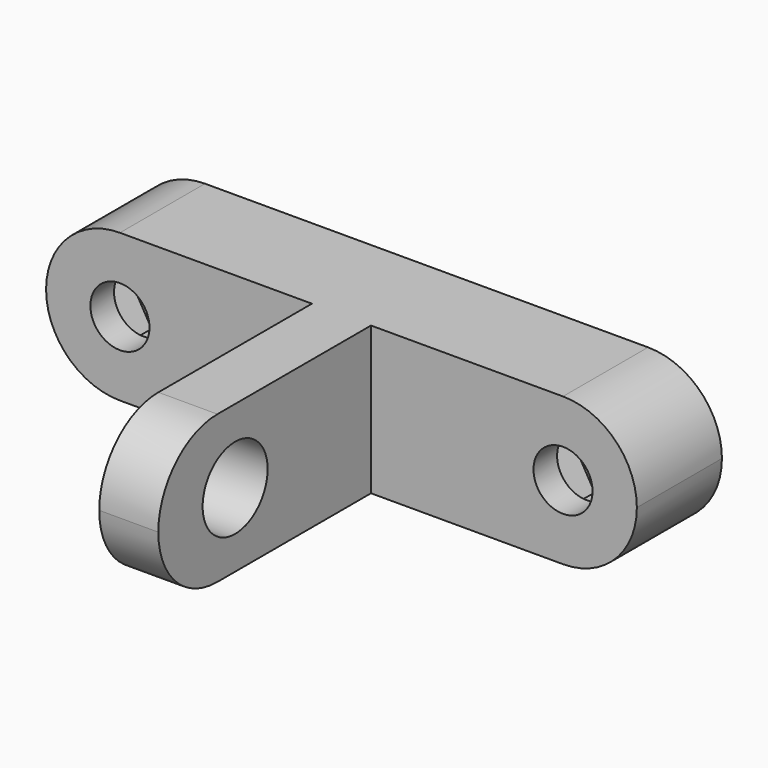
from build123d import *

# Parameters (mm, degrees)
F0_W     = 40
F0_H     = 10
F0_R     = 2
F1_DEPTH = 2
F2_W     = 40
F2_H     = 10
F3_DEPTH = 3.2
F4_START = 5.2
F4_DEPTH = 2
F5_W     = 4
F5_H     = 10
F6_DEPTH = 18
F7_R     = 2.75
F8_DEPTH = 25
F9_R     = 4.99999


# Not quite as in the source:
# - a fillet or chamfer is up to 0.001 mm smaller than in the source, because OpenCascade refuses the exact size


with BuildPart() as f1:
    # F0 (on Front) → F1 (new body)
    with BuildSketch(Plane.XZ):
        Rectangle(F0_W, F0_H)
        with Locations((-15, 0)):
            Circle(F0_R, mode=Mode.SUBTRACT)
        with Locations((15, 0)):
            Circle(F0_R, mode=Mode.SUBTRACT)
    extrude(amount=F1_DEPTH)

    # F2 (on face) → F3 (join)
    with BuildSketch(Plane.XZ.offset(2)):
        Rectangle(F2_W, F2_H)
        Polygon((-10.9585481157, 0), (-12.9792740578, -3.5), (-17.0207259422, -3.5), (-19.0414518843, 0), (-17.0207259422, 3.5), (-12.9792740578, 3.5), align=None, mode=Mode.SUBTRACT)
        Polygon((19.0414518843, 0), (17.0207259422, -3.5), (12.9792740578, -3.5), (10.9585481157, 0), (12.9792740578, 3.5), (17.0207259422, 3.5), align=None, mode=Mode.SUBTRACT)
    extrude(amount=F3_DEPTH)

    # F0 (on Front) → F4 (join)
    with BuildSketch(Plane.XZ.offset(F4_START)):
        Rectangle(F0_W, F0_H)
        with Locations((-15, 0)):
            Circle(F0_R, mode=Mode.SUBTRACT)
        with Locations((15, 0)):
            Circle(F0_R, mode=Mode.SUBTRACT)
    extrude(amount=F4_DEPTH)

    # F5 (on face) → F6 (join)
    with BuildSketch(Plane.XZ.offset(7.2)):
        Rectangle(F5_W, F5_H)
    extrude(amount=F6_DEPTH)

    # F7 (on face) → F8 (cut)
    with BuildSketch(Plane.YZ.offset(2)):
        with Locations((-18.7, 0)):
            Circle(F7_R)
    extrude(amount=-F8_DEPTH, mode=Mode.SUBTRACT)

    # F9 (radius 5 in the source; OpenCascade refuses exactly that, so slightly less here)
    f9_edges = [f1.edges().sort_by_distance(p)[0] for p in [
        (0, -25.2, 5),
        (0, -25.2, -5),
        (20, -3.6, 5),
        (20, -3.6, -5),
        (-20, -3.6, 5),
        (-20, -3.6, -5),
    ]]
    fillet(f9_edges, radius=F9_R)


solid = f1.part
